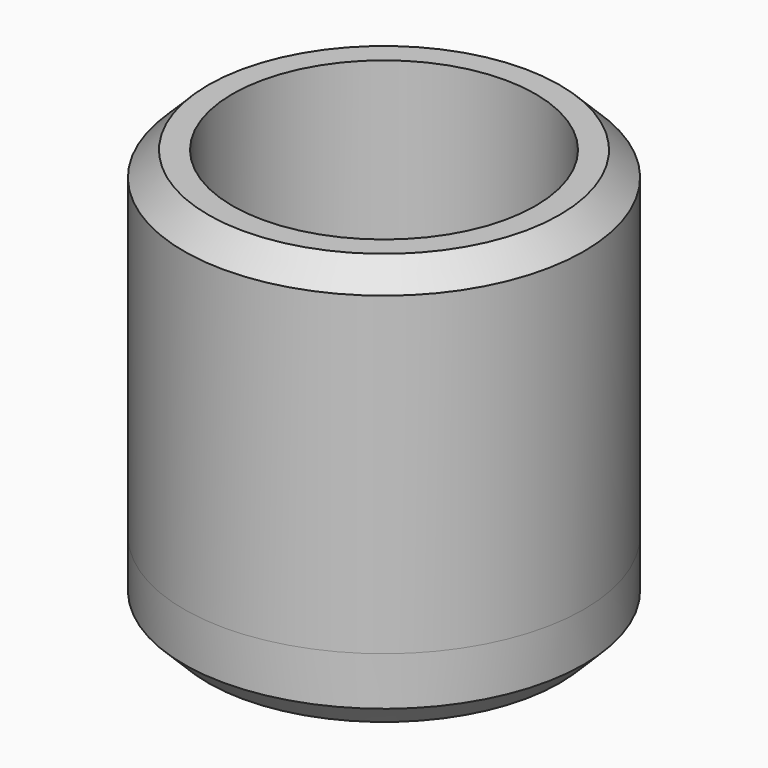
from build123d import *

# Parameters (mm, degrees)
F0_R     = 8.25
F0_R_2   = 6.25
F1_DEPTH = 11
F2_DEPTH = 3
F3_R     = 8.25
F3_R_2   = 1.5
F4_DEPTH = 3
F5_SIZE  = 1


with BuildPart() as f1:
    # F0 (on Top) → F1 (new body)
    with BuildSketch(Plane.XY):
        Circle(F0_R)
        Circle(F0_R_2, mode=Mode.SUBTRACT)
    extrude(amount=F1_DEPTH)

    # F0 (on Top) → F2 (join)
    with BuildSketch(Plane.XY):
        Circle(F0_R)
        Circle(F0_R_2, mode=Mode.SUBTRACT)
        Circle(F0_R_2)
        Polygon((2.9444863729, -1.7), (0, -3.4), (-2.9444863729, -1.7), (-2.9444863729, 1.7), (0, 3.4), (2.9444863729, 1.7), align=None, mode=Mode.SUBTRACT)
    extrude(amount=-F2_DEPTH)

    # F3 (on face) → F4 (join)
    with BuildSketch(Plane(origin=(0, 0, -3), x_dir=(1, 0, 0), z_dir=(0, 0, -1))):
        Circle(F3_R)
        Polygon((0, 3.4), (2.9444863729, 1.7), (2.9444863729, -1.7), (0, -3.4), (-2.9444863729, -1.7), (-2.9444863729, 1.7), align=None, mode=Mode.SUBTRACT)
        Polygon((2.9444863729, -1.7), (2.9444863729, 1.7), (0, 3.4), (-2.9444863729, 1.7), (-2.9444863729, -1.7), (0, -3.4), align=None)
        Circle(F3_R_2, mode=Mode.SUBTRACT)
    extrude(amount=F4_DEPTH)

    # F5
    f5_edges = [f1.edges().sort_by_distance(p)[0] for p in [
        (-8.25, 0, 11),
        (-8.25, 0, -6),
        (-1.5, 0, -6),
    ]]
    chamfer(f5_edges, length=F5_SIZE)


solid = f1.part
